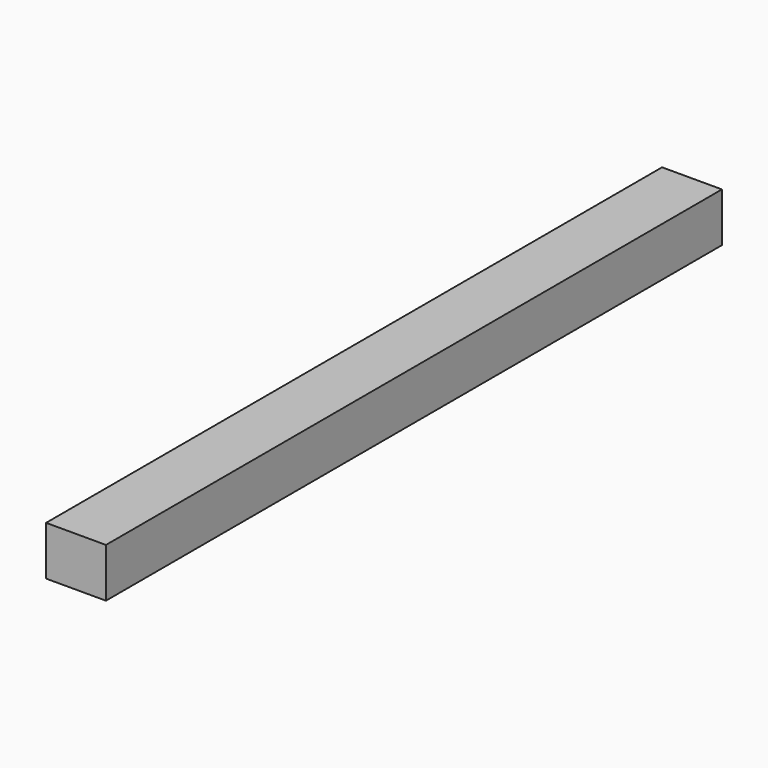
from build123d import *

# Parameters (mm, degrees)
F1_E0_TOP_W = 114.9231269956
F1_E0_TOP_H = 8.9353490621
F2_DEPTH    = 7.3296674527


with BuildPart() as f2:
    # F1_E0_top (on explicit) → F2 (new body)
    with BuildSketch(Plane(origin=(0, 0, 36.2498909235), x_dir=(0, -1, 0), z_dir=(0, 0, -1))):
        with Locations((57.4615634978, 4.467674531)):
            Rectangle(F1_E0_TOP_W, F1_E0_TOP_H)
    extrude(amount=F2_DEPTH)


solid = f2.part
